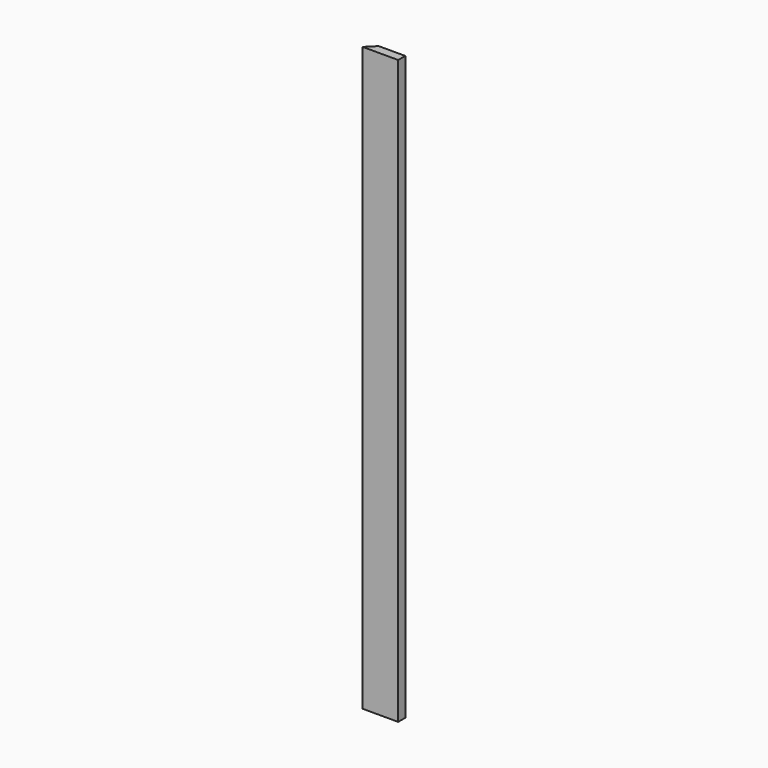
from build123d import *

# Parameters (mm, degrees)
F0_W     = 76.2
F0_H     = 19.05
F1_DEPTH = 625.475
F2_SIZE2 = 19.04999
F2_SIZE  = 19.04999


# Not quite as in the source:
# - a fillet or chamfer is up to 0.001 mm smaller than in the source, because OpenCascade refuses the exact size


with BuildPart() as f1:
    # F0 (on Top) → F1 (new body, symmetric)
    with BuildSketch(Plane.XY):
        Rectangle(F0_W, F0_H)
    extrude(amount=F1_DEPTH, both=True)

    # F2 (size 19.05 and 19.05 in the source; OpenCascade refuses exactly that, so slightly less here)
    f2_edges = [f1.edges().sort_by_distance(p)[0] for p in [
        (-38.1, 9.525, 0),
    ]]
    chamfer(f2_edges, length=F2_SIZE, length2=F2_SIZE2)


solid = f1.part
